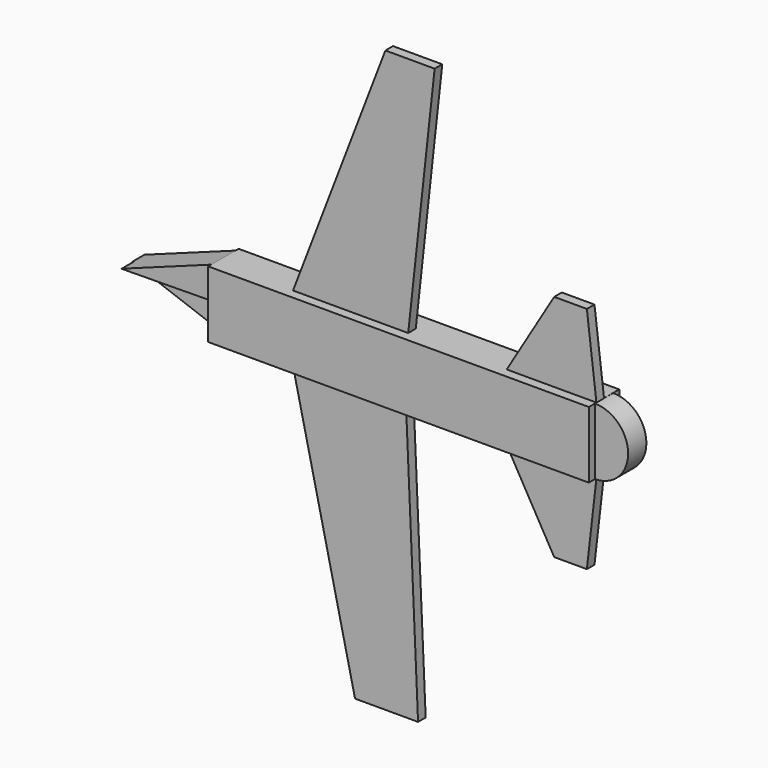
from build123d import *

# Parameters (mm, degrees)
F1_DEPTH  = 6.35
F2_DEPTH  = 6.35
F3_DEPTH  = 12.7
F4_DEPTH  = 12.7
F5_DEPTH  = 6.35
F6_DEPTH  = 6.35
F7_DEPTH  = 12.7
F8_DEPTH  = 12.7
F9_DEPTH  = 7.62
F10_DEPTH = 7.62
F12_DEPTH = 10.16
F13_DEPTH = 10.16


with BuildPart() as f1:
    # F0 (on Front) → F1 (new body)
    with BuildSketch(Plane.XZ):
        Polygon((-14.650022611, 166.190251708), (-76.259791851, 5.1223636389), (0.5617379969, 5.1223636389), (18.2250589132, 166.190251708), align=None)
    extrude(amount=F1_DEPTH)


with BuildPart() as f2:
    # F0 (on Front) → F2 (new body)
    with BuildSketch(Plane.XZ):
        Polygon((-0.804517746, -39.3276363611), (-76.259791851, -39.3276363611), (-34.8977893591, -221.2072610855), (7.1541545913, -221.2072610855), align=None)
    extrude(amount=F2_DEPTH)


with BuildPart() as f3:
    # F0 (on Front) → F3 (new body)
    with BuildSketch(Plane.XZ):
        with BuildLine():
            Line((-127.804517746, 5.1223636389), (-127.804517746, -39.3276363611))
            Line((-127.804517746, -39.3276363611), (-76.259791851, -39.3276363611))
            Line((-76.259791851, -39.3276363611), (-0.804517746, -39.3276363611))
            Line((-0.804517746, -39.3276363611), (66.3339793682, -39.3276363611))
            Line((66.3339793682, -39.3276363611), (126.195482254, -39.3276363611))
            Line((126.195482254, -39.3276363611), (126.195482254, -39.2710786657))
            ThreePointArc((126.195482254, -39.2710786657), (104.0270399495, -17.1026363611), (126.195482254, 5.0658059434))
            Line((126.195482254, 5.0658059434), (126.195482254, 5.1223636389))
            Line((126.195482254, 5.1223636389), (66.3339793682, 5.1223636389))
            Line((66.3339793682, 5.1223636389), (0.5617379969, 5.1223636389))
            Line((0.5617379969, 5.1223636389), (-76.259791851, 5.1223636389))
            Line((-76.259791851, 5.1223636389), (-127.804517746, 5.1223636389))
        make_face()
    extrude(amount=F3_DEPTH)

    # F0 (on Front) → F4 (join)
    with BuildSketch(Plane.XZ):
        with BuildLine():
            Line((-127.804517746, 5.1223636389), (-127.804517746, -39.3276363611))
            Line((-127.804517746, -39.3276363611), (-76.259791851, -39.3276363611))
            Line((-76.259791851, -39.3276363611), (-0.804517746, -39.3276363611))
            Line((-0.804517746, -39.3276363611), (66.3339793682, -39.3276363611))
            Line((66.3339793682, -39.3276363611), (126.195482254, -39.3276363611))
            Line((126.195482254, -39.3276363611), (126.195482254, -39.2710786657))
            ThreePointArc((126.195482254, -39.2710786657), (104.0270399495, -17.1026363611), (126.195482254, 5.0658059434))
            Line((126.195482254, 5.0658059434), (126.195482254, 5.1223636389))
            Line((126.195482254, 5.1223636389), (66.3339793682, 5.1223636389))
            Line((66.3339793682, 5.1223636389), (0.5617379969, 5.1223636389))
            Line((0.5617379969, 5.1223636389), (-76.259791851, 5.1223636389))
            Line((-76.259791851, 5.1223636389), (-127.804517746, 5.1223636389))
        make_face()
    extrude(amount=-F4_DEPTH)

    # F0 (on Front) → F5 (join)
    with BuildSketch(Plane.XZ):
        Polygon((126.195482254, -39.3276363611), (66.3339793682, -39.3276363611), (97.9932621121, -94.8227718472), (119.8113709688, -94.8227718472), align=None)
    extrude(amount=F5_DEPTH)

    # F0 (on Front) → F6 (join)
    with BuildSketch(Plane.XZ):
        Polygon((97.9932621121, 58.0698437989), (66.3339793682, 5.1223636389), (126.195482254, 5.1223636389), (119.8113709688, 58.0698437989), align=None)
    extrude(amount=F6_DEPTH)

    # F0 (on Front) → F7 (join)
    with BuildSketch(Plane.XZ):
        with BuildLine():
            ThreePointArc((126.195482254, 5.0658059434), (104.0270399495, -17.1026363611), (126.195482254, -39.2710786657))
            Line((126.195482254, -39.2710786657), (126.195482254, 5.0658059434))
        make_face()
    extrude(amount=F7_DEPTH)

    # F0 (on Front) → F8 (join)
    with BuildSketch(Plane.XZ):
        with BuildLine():
            ThreePointArc((126.195482254, 5.0658059434), (104.0270399495, -17.1026363611), (126.195482254, -39.2710786657))
            Line((126.195482254, -39.2710786657), (126.195482254, 5.0658059434))
        make_face()
    extrude(amount=-F8_DEPTH)

    # F0 (on Front) → F9 (join)
    with BuildSketch(Plane.XZ):
        with BuildLine():
            Line((126.195482254, 5.0658059434), (126.195482254, -39.2710786657))
            ThreePointArc((126.195482254, -39.2710786657), (141.8709381359, -32.778092243), (148.3639245586, -17.1026363611))
            ThreePointArc((148.3639245586, -17.1026363611), (141.8709381359, -1.4271804792), (126.195482254, 5.0658059434))
        make_face()
    extrude(amount=F9_DEPTH)

    # F0 (on Front) → F10 (join)
    with BuildSketch(Plane.XZ):
        with BuildLine():
            Line((126.195482254, 5.0658059434), (126.195482254, -39.2710786657))
            ThreePointArc((126.195482254, -39.2710786657), (141.8709381359, -32.778092243), (148.3639245586, -17.1026363611))
            ThreePointArc((148.3639245586, -17.1026363611), (141.8709381359, -1.4271804792), (126.195482254, 5.0658059434))
        make_face()
    extrude(amount=-F10_DEPTH)

    # F11 (on face) → F12 (join)
    with BuildSketch(Plane.XZ):
        Polygon((-127.804517746, 5.1223636389), (-187.6378862633, -16.7326647788), (-181.624352932, -16.7326647788), (-127.804517746, -16.0813909283), align=None)
    extrude(amount=F12_DEPTH)

    # F0 (on Front) → F13 (join)
    with BuildSketch(Plane.XZ):
        Polygon((-188.6507719755, -17.1026363611), (-127.804517746, -39.3276363611), (-127.804517746, 5.1223636389), align=None)
    extrude(amount=-F13_DEPTH)


solid = Compound([f1.part, f2.part, f3.part])
